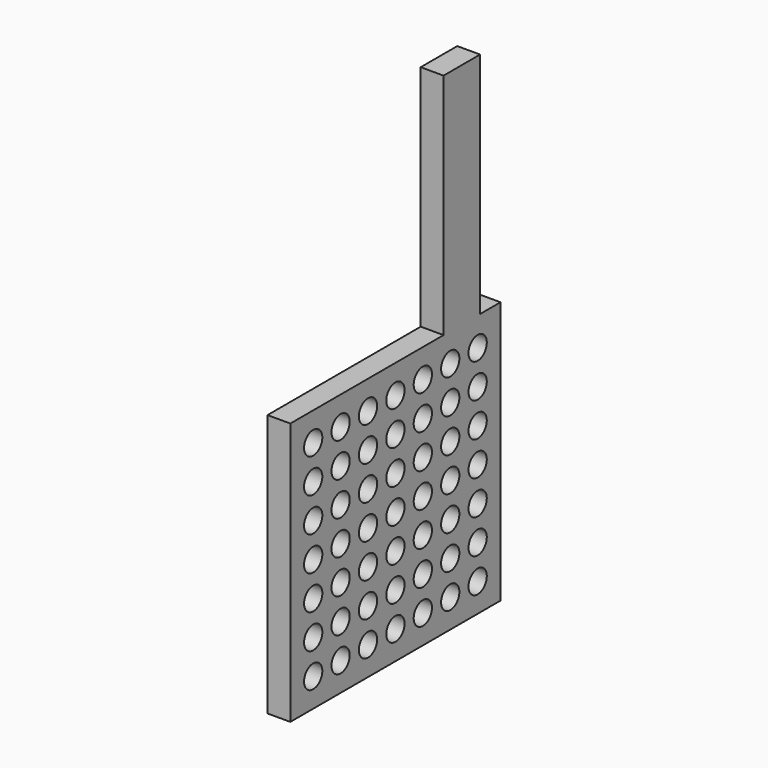
from build123d import *

# Parameters (mm, degrees)
F0_R     = 0.5
F1_DEPTH = 1


# Not quite as in the source:
# - a feature names something its author has since deleted; it is built from what else it names


with BuildPart() as f1:
    # F0 (on Right) → F1 (new body)
    with BuildSketch(Plane.YZ):
        Polygon((8.384144865, 0), (0, 0), (0, -11.5), (11.5, -11.5), (11.5, 0), (10.384144865, 0), (10.384144865, 10), (8.384144865, 10), align=None)
        with Locations((1.25, -10.249999141)):
            Circle(F0_R, mode=Mode.SUBTRACT)
        with Locations((2.75, -10.249999141)):
            Circle(F0_R, mode=Mode.SUBTRACT)
        with Locations((1.25, -8.7499995705)):
            Circle(F0_R, mode=Mode.SUBTRACT)
        with Locations((1.25, -7.25)):
            Circle(F0_R, mode=Mode.SUBTRACT)
        with Locations((2.75, -8.7499995705)):
            Circle(F0_R, mode=Mode.SUBTRACT)
        with Locations((2.75, -7.25)):
            Circle(F0_R, mode=Mode.SUBTRACT)
        with Locations((4.25, -10.249999141)):
            Circle(F0_R, mode=Mode.SUBTRACT)
        with Locations((4.25, -8.7499995705)):
            Circle(F0_R, mode=Mode.SUBTRACT)
        with Locations((4.25, -7.25)):
            Circle(F0_R, mode=Mode.SUBTRACT)
        with Locations((5.7488648942, -8.7499995705)):
            Circle(F0_R, mode=Mode.SUBTRACT)
        with Locations((1.25, -5.75)):
            Circle(F0_R, mode=Mode.SUBTRACT)
        with Locations((1.25, -4.25)):
            Circle(F0_R, mode=Mode.SUBTRACT)
        with Locations((2.75, -5.75)):
            Circle(F0_R, mode=Mode.SUBTRACT)
        with Locations((2.75, -4.25)):
            Circle(F0_R, mode=Mode.SUBTRACT)
        with Locations((1.25, -2.7500004295)):
            Circle(F0_R, mode=Mode.SUBTRACT)
        with Locations((1.25, -1.250000859)):
            Circle(F0_R, mode=Mode.SUBTRACT)
        with Locations((2.75, -2.7500004295)):
            Circle(F0_R, mode=Mode.SUBTRACT)
        with Locations((2.75, -1.250000859)):
            Circle(F0_R, mode=Mode.SUBTRACT)
        with Locations((4.25, -5.75)):
            Circle(F0_R, mode=Mode.SUBTRACT)
        with Locations((4.25, -4.25)):
            Circle(F0_R, mode=Mode.SUBTRACT)
        with Locations((4.25, -2.7500004295)):
            Circle(F0_R, mode=Mode.SUBTRACT)
        with Locations((4.25, -1.250000859)):
            Circle(F0_R, mode=Mode.SUBTRACT)
        with Locations((5.7488648942, -2.7500004295)):
            Circle(F0_R, mode=Mode.SUBTRACT)
        with Locations((5.75, -10.249999141)):
            Circle(F0_R, mode=Mode.SUBTRACT)
        with Locations((7.25, -10.249999141)):
            Circle(F0_R, mode=Mode.SUBTRACT)
        with Locations((5.75, -7.25)):
            Circle(F0_R, mode=Mode.SUBTRACT)
        with Locations((7.25, -8.7499995705)):
            Circle(F0_R, mode=Mode.SUBTRACT)
        with Locations((7.25, -7.25)):
            Circle(F0_R, mode=Mode.SUBTRACT)
        with Locations((8.75, -10.249999141)):
            Circle(F0_R, mode=Mode.SUBTRACT)
        with Locations((10.25, -10.249999141)):
            Circle(F0_R, mode=Mode.SUBTRACT)
        with Locations((8.75, -8.7499995705)):
            Circle(F0_R, mode=Mode.SUBTRACT)
        with Locations((8.75, -7.25)):
            Circle(F0_R, mode=Mode.SUBTRACT)
        with Locations((10.25, -8.7499995705)):
            Circle(F0_R, mode=Mode.SUBTRACT)
        with Locations((10.25, -7.25)):
            Circle(F0_R, mode=Mode.SUBTRACT)
        with Locations((5.75, -5.75)):
            Circle(F0_R, mode=Mode.SUBTRACT)
        with Locations((5.75, -4.25)):
            Circle(F0_R, mode=Mode.SUBTRACT)
        with Locations((7.25, -5.75)):
            Circle(F0_R, mode=Mode.SUBTRACT)
        with Locations((7.25, -4.25)):
            Circle(F0_R, mode=Mode.SUBTRACT)
        with Locations((5.75, -1.250000859)):
            Circle(F0_R, mode=Mode.SUBTRACT)
        with Locations((7.25, -2.7500004295)):
            Circle(F0_R, mode=Mode.SUBTRACT)
        with Locations((7.25, -1.250000859)):
            Circle(F0_R, mode=Mode.SUBTRACT)
        with Locations((8.75, -5.75)):
            Circle(F0_R, mode=Mode.SUBTRACT)
        with Locations((8.75, -4.25)):
            Circle(F0_R, mode=Mode.SUBTRACT)
        with Locations((10.25, -5.75)):
            Circle(F0_R, mode=Mode.SUBTRACT)
        with Locations((10.25, -4.25)):
            Circle(F0_R, mode=Mode.SUBTRACT)
        with Locations((8.75, -2.7500004295)):
            Circle(F0_R, mode=Mode.SUBTRACT)
        with Locations((8.75, -1.250000859)):
            Circle(F0_R, mode=Mode.SUBTRACT)
        with Locations((10.25, -2.7500004295)):
            Circle(F0_R, mode=Mode.SUBTRACT)
        with Locations((10.25, -1.250000859)):
            Circle(F0_R, mode=Mode.SUBTRACT)
    extrude(amount=F1_DEPTH)


solid = f1.part
